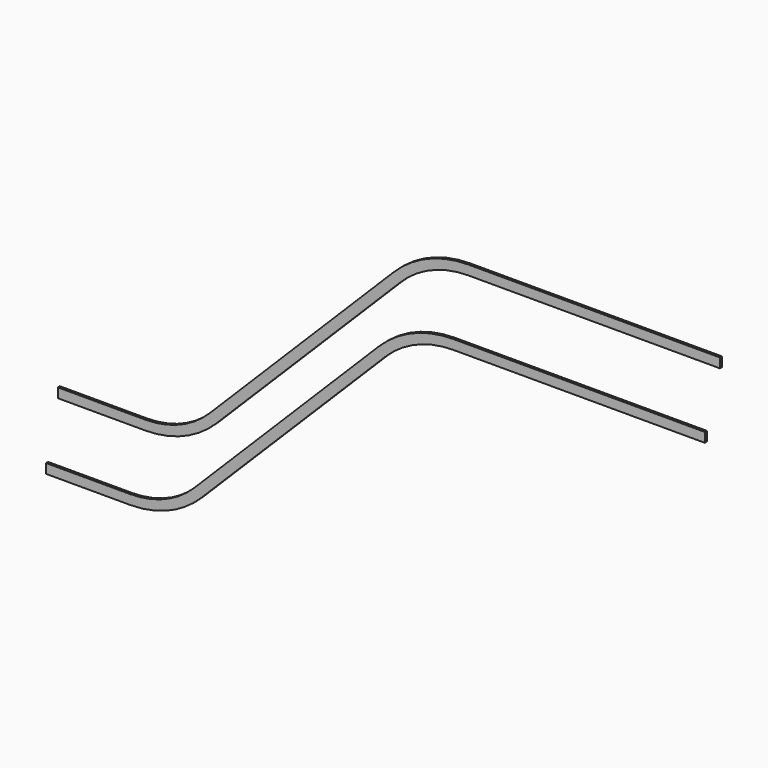
from build123d import *

# Parameters (mm, degrees)
F1_DEPTH = 10


# Not quite as in the source:
# - a feature names something its author has since deleted; it is built from what else it names


with BuildPart() as f1:
    # F0 (on Front) → F1 (new body)
    with BuildSketch(Plane.XZ):
        with BuildLine():
            Line((897.5679823155, 1139.4882925322), (807.5679823155, 1049.4882925322))
            Line((807.5679823155, 1049.4882925322), (805.0931085813, 1051.9631662664))
            Line((805.0931085813, 1051.9631662664), (163.7222586828, 410.5923163679))
            ThreePointArc((163.7222586828, 410.5923163679), (46.2810064095, 332.1205803884), (-92.2503961067, 304.5649711575))
            Line((-92.2503961067, 304.5649711575), (-105.134062469, 304.5649711575))
            Line((-105.134062469, 304.5649711575), (-440, 304.5649711575))
            Line((-440, 304.5649711575), (-440, 266.5649711575))
            Line((-440, 266.5649711575), (-92.2503961067, 266.5649711575))
            ThreePointArc((-92.2503961067, 266.5649711575), (60.8229768393, 297.0131581529), (190.5923163679, 383.7222586828))
            Line((190.5923163679, 383.7222586828), (921.9631662664, 1115.0931085813))
            ThreePointArc((921.9631662664, 1115.0931085813), (1045.5684621674, 1197.683526836), (1191.3708498985, 1226.6854249492))
            Line((1191.3708498985, 1226.6854249492), (2191.3708498985, 1226.6854249492))
            Line((2191.3708498985, 1226.6854249492), (2191.3708498985, 1245.6854249492))
            Line((2191.3708498985, 1245.6854249492), (2191.3708498985, 1261.1854249041))
            Line((2191.3708498985, 1261.1854249041), (1191.3647249172, 1261.1854249041))
            ThreePointArc((1191.3647249172, 1261.1854249041), (1032.3630543827, 1229.5561987328), (897.5679823155, 1139.4882925322))
        make_face()
        Polygon((805.0931085813, 1051.9631662664), (807.5679823155, 1049.4882925322), (897.5679823155, 1139.4882925322), (895.0931085813, 1141.9631662664), align=None)
        with BuildLine():
            Line((895.0931085813, 1141.9631662664), (897.5679823155, 1139.4882925322))
            ThreePointArc((897.5679823155, 1139.4882925322), (1032.3630543827, 1229.5561987328), (1191.3647249172, 1261.1854249041))
            Line((1191.3647249172, 1261.1854249041), (2191.3708498985, 1261.1854249041))
            Line((2191.3708498985, 1261.1854249041), (2191.3708498985, 1264.6854249492))
            Line((2191.3708498985, 1264.6854249492), (1191.3708498985, 1264.6854249492))
            ThreePointArc((1191.3708498985, 1264.6854249492), (1191.3677874079, 1264.685424938), (1191.3647249172, 1264.6854249045))
            ThreePointArc((1191.3647249172, 1264.6854249045), (1031.0236623694, 1232.7897770967), (895.0931085813, 1141.9631662664))
        make_face()
    extrude(amount=F1_DEPTH)


with BuildPart() as f1b:
    # F0 (on Front) → F1, piece 2 (new body)
    with BuildSketch(Plane.XZ):
        with BuildLine():
            Line((837.5679823155, 859.4882925322), (835.0931085813, 861.9631662664))
            Line((835.0931085813, 861.9631662664), (103.7222586828, 130.5923163679))
            ThreePointArc((103.7222586828, 130.5923163679), (-13.7189935905, 52.1205803884), (-152.2503961067, 24.5649711575))
            Line((-152.2503961067, 24.5649711575), (-486.5649711575, 24.5649711575))
            Line((-486.5649711575, 24.5649711575), (-486.5649711575, -13.4350288425))
            Line((-486.5649711575, -13.4350288425), (-152.2503961067, -13.4350288425))
            ThreePointArc((-152.2503961067, -13.4350288425), (-80.9692466878, -7.0325361232), (-11.9699824698, 11.9699824698))
            ThreePointArc((-11.9699824698, 11.9699824698), (64.2280439518, 50.206405056), (130.5923163679, 103.7222586828))
            Line((130.5923163679, 103.7222586828), (861.9631662664, 835.0931085813))
            Line((861.9631662664, 835.0931085813), (848.5281374239, 848.5281374239))
            Line((848.5281374239, 848.5281374239), (837.5679823155, 859.4882925322))
        make_face()
        with BuildLine():
            ThreePointArc((1131.3708498985, 984.6854249492), (971.0264917375, 952.7909490715), (835.0931085813, 861.9631662664))
            Line((835.0931085813, 861.9631662664), (837.5679823155, 859.4882925322))
            Line((837.5679823155, 859.4882925322), (848.5281374239, 848.5281374239))
            Line((848.5281374239, 848.5281374239), (861.9631662664, 835.0931085813))
            ThreePointArc((861.9631662664, 835.0931085813), (985.5684621674, 917.683526836), (1131.3708498985, 946.6854249492))
            Line((1131.3708498985, 946.6854249492), (1131.3708498985, 965.6854249492))
            Line((1131.3708498985, 965.6854249492), (1131.3708498985, 984.6854249492))
        make_face()
        Polygon((2131.3708498985, 984.6854249492), (1131.3708498985, 984.6854249492), (1131.3708498985, 965.6854249492), (1131.3708498985, 946.6854249492), (2131.3708498985, 946.6854249492), align=None)
    extrude(amount=F1_DEPTH)


solid = Compound([f1.part, f1b.part])
